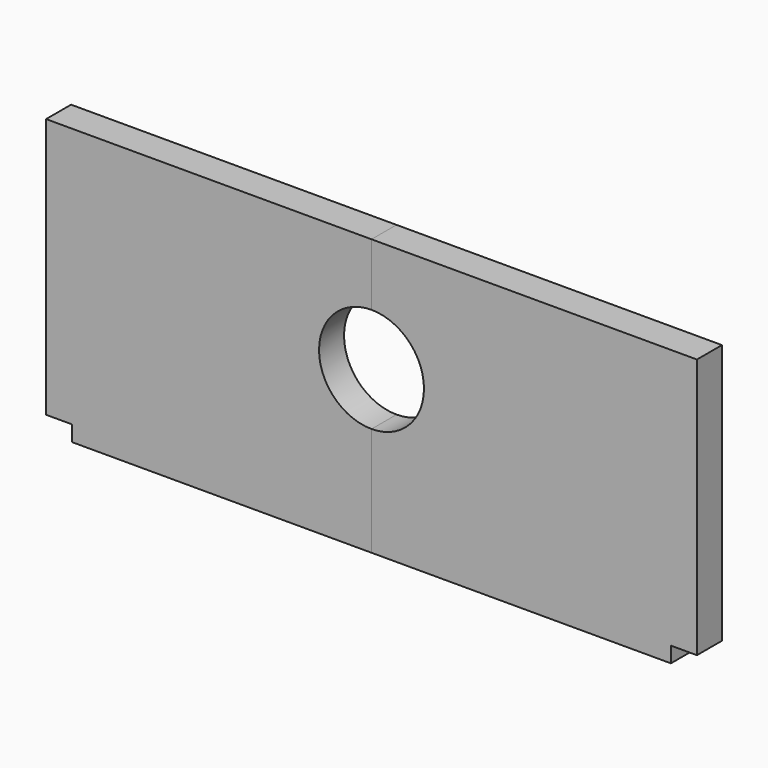
from build123d import *
from build123d import SkipClean  # not in build123d's __all__

# Parameters (mm, degrees)
F1_DEPTH = 6


with BuildPart() as f1:
    # F0 (on Front) → F1 (new body)
    with BuildSketch(Plane.XZ):
        with BuildLine():
            Line((-57.5, 0), (0, 0))
            Line((0, 0), (0, 20.925))
            ThreePointArc((0, 20.925), (-10.075, 31), (0, 41.075))
            Line((0, 41.075), (0, 53))
            Line((0, 53), (-62.5, 53))
            Line((-62.5, 53), (-62.5, 3))
            Line((-62.5, 3), (-57.5, 3))
            Line((-57.5, 3), (-57.5, 0))
        make_face()
    extrude(amount=F1_DEPTH)

    # F2: F1 across face


with BuildPart() as f1_1:
    add(f1.part, clean=False)
    with SkipClean():  # cleaning this boolean's faces spoils the solid; the shape is the same uncleaned
        add(f1.part.mirror(Plane(origin=(0, -3, 47.0375), x_dir=(0, 1, 0), z_dir=(1, 0, 0))), clean=False)


solid = f1_1.part
